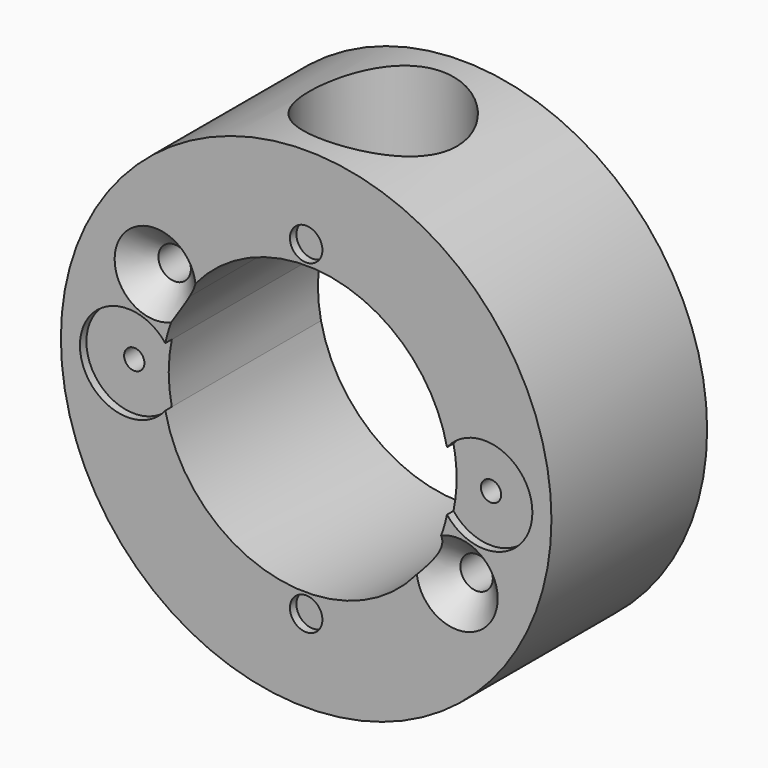
from build123d import *

# Parameters (mm, degrees)
F0_R     = 30.25
F0_R_2   = 2
F1_DEPTH = 24
F0_R_3   = 1.25
F2_DEPTH = 23
F5_R     = 9.125
F5_R_2   = 8
F6_DEPTH = 25
F7_DEPTH = 15


# Not quite as in the source:
# - a fillet or chamfer that OpenCascade refuses, or shapes differently, is made with other operations: its cross-section is extruded or revolved along the edge and cut away or added


with BuildPart() as f1:
    # F0 (on Front) → F1 (new body)
    with BuildSketch(Plane.XZ):
        Circle(F0_R)
        with Locations((0, -20.07)):
            Circle(F0_R_2, mode=Mode.SUBTRACT)
        with Locations((18.6195461814, -10.75)):
            Circle(F0_R_2, mode=Mode.SUBTRACT)
        with BuildLine():
            ThreePointArc((-16.6195461814, 10.75), (-16.6876945288, 10.2323619098), (-16.8874953738, 9.75))
            ThreePointArc((-16.8874953738, 9.75), (-20.5513978339, 11.2676380902), (-16.6195461814, 10.75))
        make_face(mode=Mode.SUBTRACT)
        with BuildLine():
            ThreePointArc((8.875, 15.3719509172), (14.3703479176, 10.4190019065), (17.369375, 3.6561334917))
            ThreePointArc((17.369375, 3.6561334917), (23.9351114309, 5.5736293158), (27.9, 0))
            ThreePointArc((27.9, 0), (23.9351114309, -5.5736293158), (17.369375, -3.6561334917))
            ThreePointArc((17.369375, -3.6561334917), (0, -17.75), (-17.369375, -3.6561334917))
            ThreePointArc((-17.369375, -3.6561334917), (-27.9, 0), (-17.369375, 3.6561334917))
            ThreePointArc((-17.369375, 3.6561334917), (-16.5773263107, 6.3446632999), (-15.3719509172, 8.875))
            ThreePointArc((-15.3719509172, 8.875), (-4.5940380506, 17.1451834166), (8.875, 15.3719509172))
        make_face(mode=Mode.SUBTRACT)
        with Locations((0, 20.07)):
            Circle(F0_R_2, mode=Mode.SUBTRACT)
    extrude(amount=F1_DEPTH)

    # F0 (on Front) → F2 (join)
    with BuildSketch(Plane.XZ):
        with BuildLine():
            ThreePointArc((-17.369375, 3.6561334917), (-27.9, 0), (-17.369375, -3.6561334917))
            ThreePointArc((-17.369375, -3.6561334917), (-17.75, 0), (-17.369375, 3.6561334917))
        make_face()
        with Locations((-22, 0)):
            Circle(F0_R_3, mode=Mode.SUBTRACT)
        with Locations((0, 20.07)):
            Circle(F0_R_2)
        with BuildLine():
            ThreePointArc((17.369375, 3.6561334917), (17.6545873111, 1.8379463744), (17.75, 0))
            ThreePointArc((17.75, 0), (17.6545873111, -1.8379463744), (17.369375, -3.6561334917))
            ThreePointArc((17.369375, -3.6561334917), (23.9351114309, -5.5736293158), (27.9, 0))
            ThreePointArc((27.9, 0), (23.9351114309, 5.5736293158), (17.369375, 3.6561334917))
        make_face()
        with Locations((22, 0)):
            Circle(F0_R_3, mode=Mode.SUBTRACT)
        with Locations((0, -20.07)):
            Circle(F0_R_2)
    extrude(amount=F2_DEPTH)

    # F3: chamfer of 3 on 2 edges, made by hand

    # F3_s1 → F3_t2 (revolve, cut)
    with BuildSketch(Plane.XY.offset(10.75)):
        Polygon((-13.6195461814, -24), (-16.6195461814, -21), (-16.6195461814, -24), align=None)
    revolve(axis=Axis((-18.6195461814, -24, 10.75), (0, -1, 0)), mode=Mode.SUBTRACT)

    # F3_s3 → F3_t4 (revolve, cut)
    with BuildSketch(Plane.XY.offset(-10.75)):
        Polygon((23.6195461814, -24), (20.6195461814, -21), (20.6195461814, -24), align=None)
    revolve(axis=Axis((18.6195461814, -24, -10.75), (0, -1, 0)), mode=Mode.SUBTRACT)

    # F5 (on offset) → F6 (cut)
    with BuildSketch(Plane.XY.offset(18.75)):
        with Locations((0, -12.125)):
            Circle(F5_R)
        with Locations((0, -12.125)):
            Circle(F5_R_2, mode=Mode.SUBTRACT)
    extrude(amount=F6_DEPTH, mode=Mode.SUBTRACT)

    # F5 (on offset) → F7 (cut, symmetric)
    with BuildSketch(Plane.XY.offset(18.75)):
        with Locations((0, -12.125)):
            Circle(F5_R_2)
    extrude(amount=F7_DEPTH, both=True, mode=Mode.SUBTRACT)


solid = f1.part
